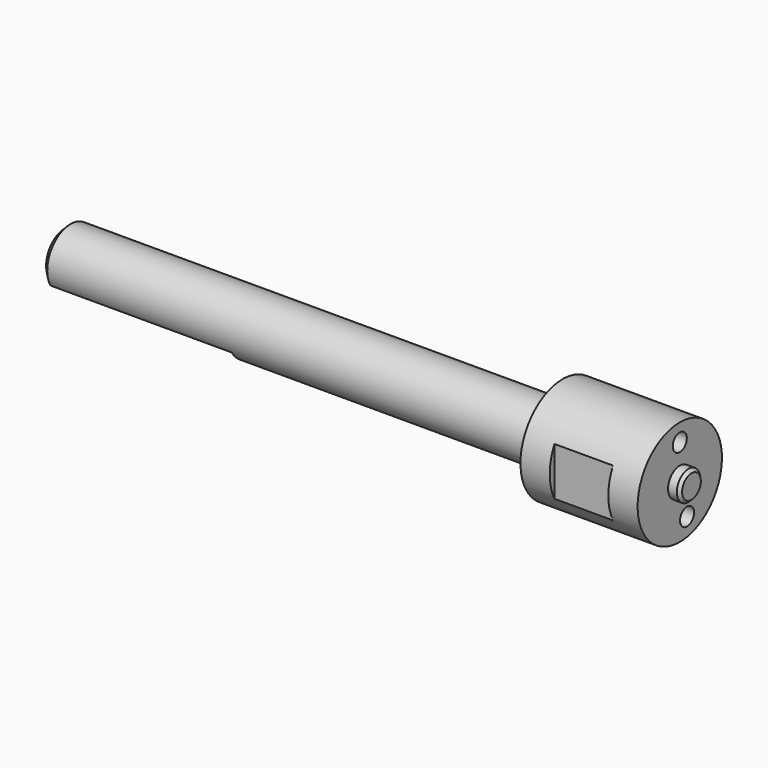
from build123d import *

# Parameters (mm, degrees)
F0_W     = 1.5
F0_H     = 2.5
F0_W_2   = 84
F0_H_2   = 5
F0_W_3   = 6
F0_H_3   = 1.23
F0_H_4   = 0.27
F3_DEPTH = 32
F4_W     = 10
F4_H     = 1
F5_DEPTH = 12.5
F8_D     = 3
F8_DEPTH = 6
F8_TIP   = 0.9012909285


# Not quite as in the source:
# - ends of sketch curves that miss each other by under 0.0002 mm in the source are joined


with BuildPart() as f1:
    # F0 (on Front) → F1 (revolve)
    with BuildSketch(Plane.XZ):
        with Locations((0.75, 1.25)):
            Rectangle(F0_W, F0_H)
        Polygon((-10, 0), (-5, 0), (-5, 4.123106), align=None)
        Polygon((-8.210141, 6), (-7.5, 6), (-7.5, 7.23), align=None)
        Polygon((-15, 0), (-10, 0), (-15, 4.123106), align=None)
        with Locations((-62, 2.5)):
            Rectangle(F0_W_2, F0_H_2)
        Polygon((0, 0), (0, 2.5), (0, 4.5), (-6, 4.5), (-6.467654, 4.77), (-7.5, 4.77), (-8.210141, 6), (-7.5, 7.23), (-6.467654, 7.23), (-6, 7.5), (0, 7.5), (0, 9), (-20, 9), (-20, 5), (-20, 0), (-15, 0), (-15, 4.123106), (-5, 4.123106), (-5, 0), align=None)
        Polygon((-15, 4.123106), (-9.9999998364, 3.651e-07), (-5, 4.123106), align=None)
        with Locations((-3, 6.615)):
            Rectangle(F0_W_3, F0_H_3)
        Polygon((2, 2), (1.5, 2.5), (1.5, 0), (2, 0), align=None)
        with Locations((-3, 5.385)):
            Rectangle(F0_W_3, F0_H_3)
        Polygon((-7.5, 6), (-6, 6), (-6, 7.23), (-6.467654, 7.23), (-7.5, 7.23), align=None)
        Polygon((-6.467654, 4.77), (-6, 4.77), (-6, 6), (-7.5, 6), (-7.5, 4.77), align=None)
        Polygon((-8.210141, 6), (-7.5, 4.77), (-7.5, 6), align=None)
        with Locations((-3, 7.365)):
            Rectangle(F0_W_3, F0_H_4)
        with Locations((-3, 4.635)):
            Rectangle(F0_W_3, F0_H_4)
        Polygon((-6.467654, 4.77), (-6, 4.5), (-6, 4.77), align=None)
        Polygon((-6.467654, 7.23), (-6, 7.23), (-6, 7.5), align=None)
        Polygon((-105, 0), (-104, 0), (-104, 5), (-105, 4), align=None)
    revolve(axis=Axis((-53, 0, 0), (-1, 0, 0)))

    # F2 (on face) → F3 (cut)
    with BuildSketch(Plane(origin=(-105, 0, 0), x_dir=(0, -1, 0), z_dir=(-1, 0, 0))):
        with BuildLine():
            Line((-3.1224989992, -2.5), (-4.330127, -2.5))
            ThreePointArc((-4.3301270142, -2.5000000082), (0, -5), (4.3301270142, -2.5000000082))
            Line((4.330127, -2.5), (3.1224989992, -2.5))
            ThreePointArc((3.1224989992, -2.5), (0, -4), (-3.1224989992, -2.5))
        make_face()
        with BuildLine():
            Line((3.1224989992, -2.5), (-3.1224989992, -2.5))
            ThreePointArc((-3.1224989992, -2.5), (0, -4), (3.1224989992, -2.5))
        make_face()
    extrude(amount=-F3_DEPTH, mode=Mode.SUBTRACT)

    # F4 (on Top) → F5 (cut, symmetric)
    with BuildSketch(Plane.XY):
        with Locations((-10, -8.5)):
            Rectangle(F4_W, F4_H)
        with Locations((-10, 8.5)):
            Rectangle(F4_W, F4_H)
    extrude(amount=F5_DEPTH, both=True, mode=Mode.SUBTRACT)

    # F8
    with Locations(Plane.YZ):
        with Locations((0, 6), (1.552915, -5.795555)):
            Hole(F8_D / 2, depth=F8_DEPTH)
            with Locations((0, 0, -(F8_DEPTH + F8_TIP / 2))):  # 118° drill point
                Cone(0, F8_D / 2, F8_TIP, mode=Mode.SUBTRACT)


solid = f1.part
